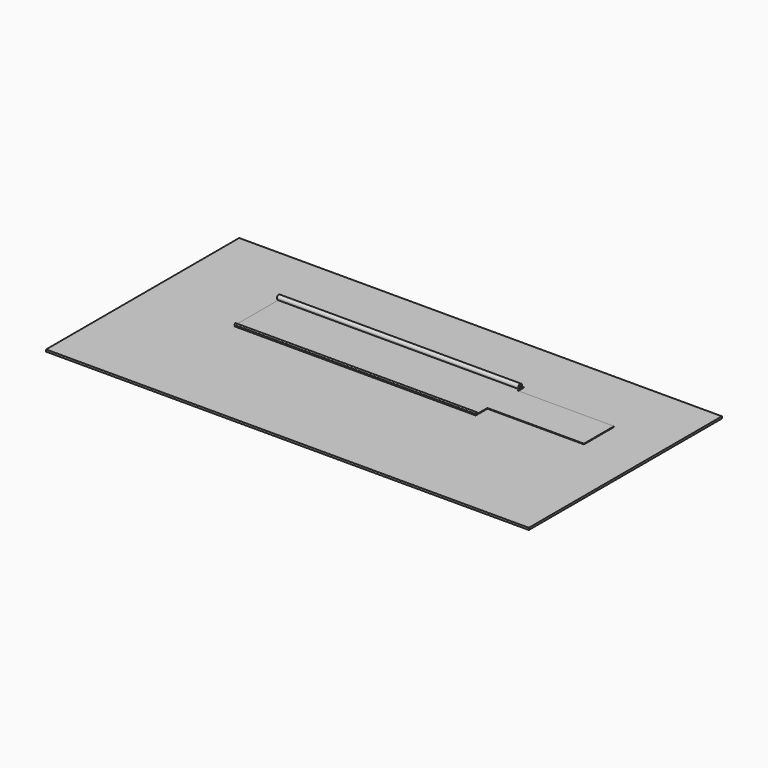
from build123d import *

# Parameters (mm, degrees)
F0_W      = 1828.8
F0_H      = 914.4
F2_DEPTH  = 7.62
F3_W      = 365.76
F3_H      = 142.6814980805
F4_DEPTH  = 7.62
F7_R      = 3.1328282943
F7_R_2    = 1.8062049827
F8_DEPTH  = 914.4
F10_R     = 8.7445702097
F10_R_2   = 4.7827305273
F11_DEPTH = 914.4


# Not quite as in the source:
# - the program builds the solid bodies; features that only make, move or delete a surface that nothing else refers to are left out


with BuildPart() as f2:
    # F0 (on Top) → F2 (new body)
    with BuildSketch(Plane.XY):
        with Locations((773.7635708094, 402.5332610428)):
            Rectangle(F0_W, F0_H)
    extrude(amount=-F2_DEPTH)


with BuildPart() as f4:
    # F3 (on Top) → F4 (new body)
    with BuildSketch(Plane.XY):
        Polygon((87.4297803879, 78.6388413668), (-826.9702196121, 78.6388413668), (-826.9702196121, -149.9611586332), (87.4297803879, -149.9611586332), (87.4297803879, -94.6356877685), (87.4297803879, 48.045810312), align=None)
        with Locations((270.3097803879, -23.2949387282)):
            Rectangle(F3_W, F3_H)
    extrude(amount=-F4_DEPTH)


with BuildPart() as f4_1:
    # F5: moved
    add(f4.part.moved(Location((1028.7, 558.8, 2.54))))

    # F7 (on offset) → F8 (join, through all)
    with BuildSketch(Plane.YZ.offset(1116.1297803879)):
        with Locations((413.2940471172, 5.6728282943)):
            Circle(F7_R)
        with Locations((413.2940471172, 5.6728282943)):
            Circle(F7_R_2, mode=Mode.SUBTRACT)
    extrude(amount=-F8_DEPTH)

    # F10 (on offset) → F11 (join, through all)
    with BuildSketch(Plane.YZ.offset(1116.1297803879)):
        with Locations((619.2727088928, 11.2845702097)):
            Circle(F10_R)
        with Locations((619.2727088928, 11.2845702097)):
            Circle(F10_R_2, mode=Mode.SUBTRACT)
    extrude(amount=-F11_DEPTH)


solid = Compound([f2.part, f4_1.part])
